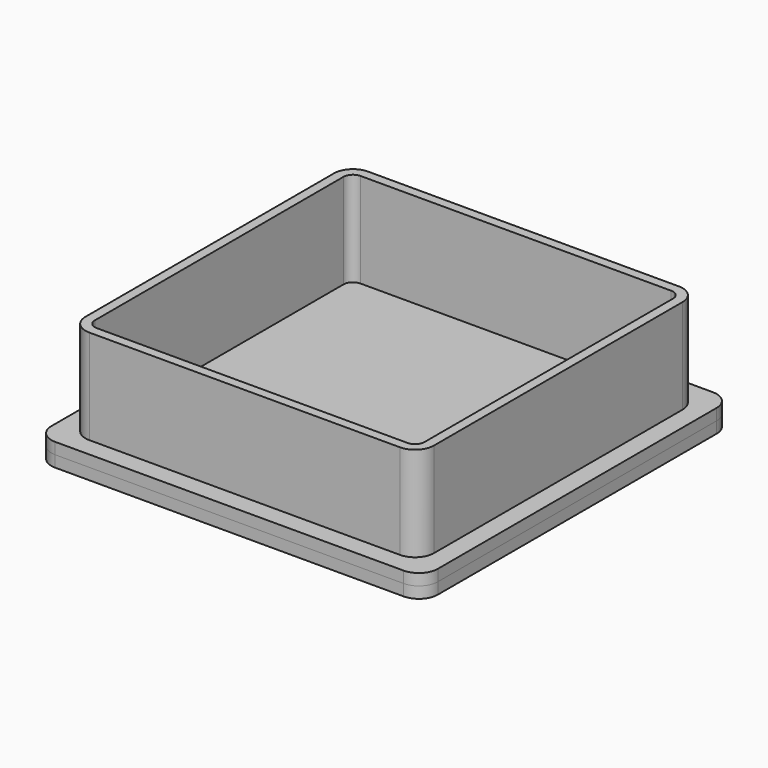
from build123d import *

# Parameters (mm, degrees)
F0_W      = 102
F0_H      = 102
F1_DEPTH  = 3
F2_R      = 5
F3_R      = 5
F4_W      = 92
F4_H      = 92
F5_DEPTH  = 28
F6_R      = 5
F7_R      = 5
F8_T      = -2.5
F9_DEPTH  = 3
F10_DEPTH = 0.5


# Not quite as in the source:
# - an extrude ends at something that could not be found from the text; its depth is read off the source's solid


with BuildPart() as f1:
    # F0 (on Top) → F1 (new body)
    with BuildSketch(Plane.XY):
        Rectangle(F0_W, F0_H)
    extrude(amount=F1_DEPTH)

    # F2
    f2_edges = [f1.edges().sort_by_distance(p)[0] for p in [
        (-51, -51, 1.5),
        (51, -51, 1.5),
        (51, 51, 1.5),
    ]]
    fillet(f2_edges, radius=F2_R)

    # F3
    f3_edges = [f1.edges().sort_by_distance(p)[0] for p in [
        (-51, 51, 1.5),
    ]]
    fillet(f3_edges, radius=F3_R)

    # F4 (on face) → F5 (join)
    with BuildSketch(Plane.XY.offset(3)):
        Rectangle(F4_W, F4_H)
    extrude(amount=F5_DEPTH)

    # F6
    f6_edges = [f1.edges().sort_by_distance(p)[0] for p in [
        (-46, -46, 17),
    ]]
    fillet(f6_edges, radius=F6_R)

    # F7
    f7_edges = [f1.edges().sort_by_distance(p)[0] for p in [
        (46, -46, 17),
        (46, 46, 17),
        (-46, 46, 17),
    ]]
    fillet(f7_edges, radius=F7_R)

    # F8
    f8_openings = [f1.faces().sort_by_distance(p)[0] for p in [
        (0, 0, 31),
    ]]
    offset(amount=F8_T, openings=f8_openings, kind=Kind.INTERSECTION)

    # F9 (add): faces of the model
    f9_faces = [f1.faces().sort_by_distance(p)[0] for p in [
        (-47.4424978336, 0, 3),
        (0, 0, 2.5),
    ]]
    extrude(f9_faces, amount=F9_DEPTH)

    # F10 (add, through all): a face of the model
    f10_faces = [f1.faces().sort_by_distance(p)[0] for p in [
        (0, 0, 5.5),
    ]]
    extrude(f10_faces, amount=F10_DEPTH)


solid = f1.part
